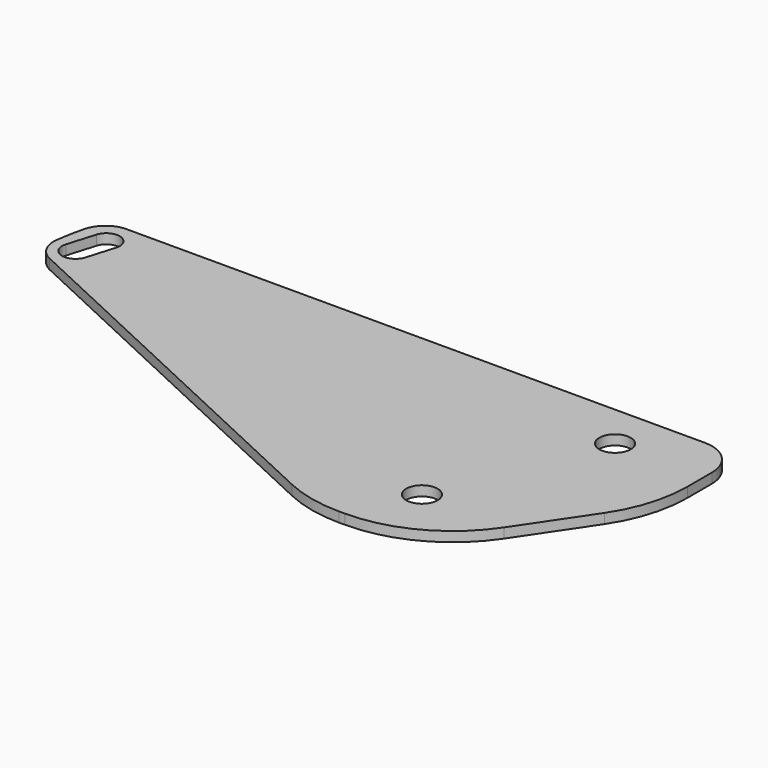
from build123d import *

# Parameters (mm, degrees)
F0_R     = 1.75
F1_DEPTH = 1.1
F2_R     = 4
F3_R     = 30
F4_R     = 15
F5_R     = 3


with BuildPart() as f1:
    # F0 (on Top) → F1 (new body)
    with BuildSketch(Plane.XY):
        Polygon((-70.716745456, 22.3987678723), (-22.682432743, 0), (-10.682432743, 0), (1.4415796787, 18), (1.4415796787, 30), (-69.2492423021, 30), (-70.4260300789, 26.0807510217), align=None)
        with Locations((-15.682432743, 7)):
            Circle(F0_R, mode=Mode.SUBTRACT)
        with BuildLine():
            Line((-69.3496626194, 24.449523286), (-68.4150438499, 27.5622371752))
            ThreePointArc((-68.4150438499, 27.5622371752), (-66.5470441613, 28.5675118458), (-65.5417694907, 26.6995121572))
            Line((-65.5417694907, 26.6995121572), (-66.4763882602, 23.586798268))
            ThreePointArc((-66.4763882602, 23.586798268), (-68.3443879488, 22.5815235974), (-69.3496626194, 24.449523286))
        make_face(mode=Mode.SUBTRACT)
        with Locations((-8.5584203213, 24.9999999582)):
            Circle(F0_R, mode=Mode.SUBTRACT)
    extrude(amount=F1_DEPTH)

    # F2
    f2_edges = [f1.edges().sort_by_distance(p)[0] for p in [
        (1.44158, 30, 0.55),
    ]]
    fillet(f2_edges, radius=F2_R)

    # F3
    f3_edges = [f1.edges().sort_by_distance(p)[0] for p in [
        (-70.42603, 26.080751, 0.55),
    ]]
    fillet(f3_edges, radius=F3_R)

    # F4
    f4_edges = [f1.edges().sort_by_distance(p)[0] for p in [
        (-22.682433, 0, 0.55),
        (1.44158, 18, 0.55),
        (-10.682433, 0, 0.55),
    ]]
    fillet(f4_edges, radius=F4_R)

    # F5
    f5_edges = [f1.edges().sort_by_distance(p)[0] for p in [
        (-69.249242, 30, 0.55),
        (-70.716745, 22.398768, 0.55),
    ]]
    fillet(f5_edges, radius=F5_R)


solid = f1.part
